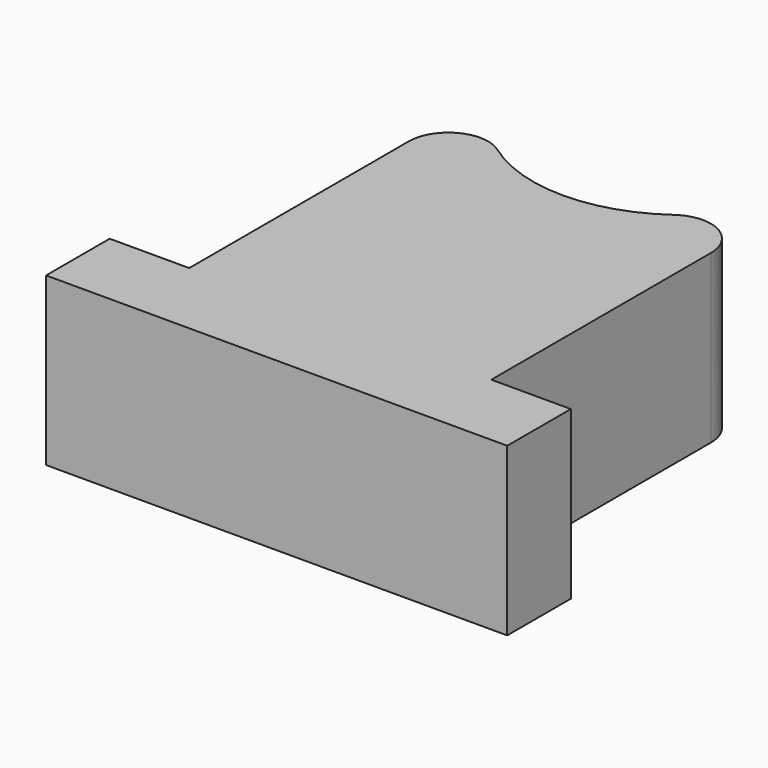
from build123d import *

# Parameters (mm, degrees)
F1_DEPTH = 2.1
F2_F1_R  = 0.5
F2_F2_R  = 0.5


with BuildPart() as f1:
    # F0 (on Top) → F1 (new body)
    with BuildSketch(Plane.XY):
        with BuildLine():
            Line((-3.9, 0.7333275447), (-3.9, -0.2666724553))
            Line((-3.9, -0.2666724553), (1.9, -0.2666724553))
            Line((1.9, -0.2666724553), (1.9, 0.7333275447))
            Line((1.9, 0.7333275447), (0.9, 0.7333275447))
            Line((0.9, 0.7333275447), (0.9, 6.1333275447))
            ThreePointArc((0.9, 6.1333275447), (-1, 4.2333275447), (-2.9, 6.1333275447))
            Line((-2.9, 6.1333275447), (-2.9, 0.7333275447))
            Line((-2.9, 0.7333275447), (-3.9, 0.7333275447))
        make_face()
    extrude(amount=F1_DEPTH)

    # F2: fillet of radius 0.5 on 2 edges, made by hand

    # F2_f1
    f2_f1_edges = [f1.edges().sort_by_distance(p)[0] for p in [
        (-2.9, 6.1333275447, 1.05),
    ]]
    fillet(f2_f1_edges, radius=F2_F1_R)

    # F2_f2
    f2_f2_edges = [f1.edges().sort_by_distance(p)[0] for p in [
        (0.9, 6.1333275447, 1.05),
    ]]
    fillet(f2_f2_edges, radius=F2_F2_R)


solid = f1.part
